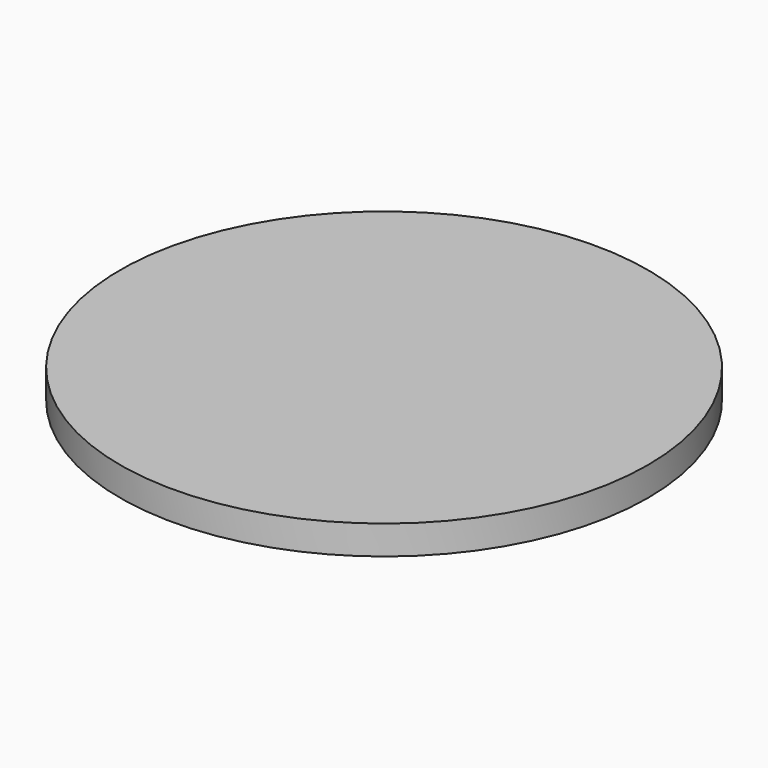
from build123d import *

# Parameters (mm, degrees)
F2_R     = 45.5
F3_DEPTH = 5


# Not quite as in the source:
# - the program builds the solid bodies; features that only make, move or delete a surface that nothing else refers to are left out


with BuildPart() as f3:
    # F2 (on Top) → F3 (new body)
    with BuildSketch(Plane.XY):
        with Locations((-46.3043488562, 17.1195659786)):
            Circle(F2_R)
    extrude(amount=F3_DEPTH)


solid = f3.part
